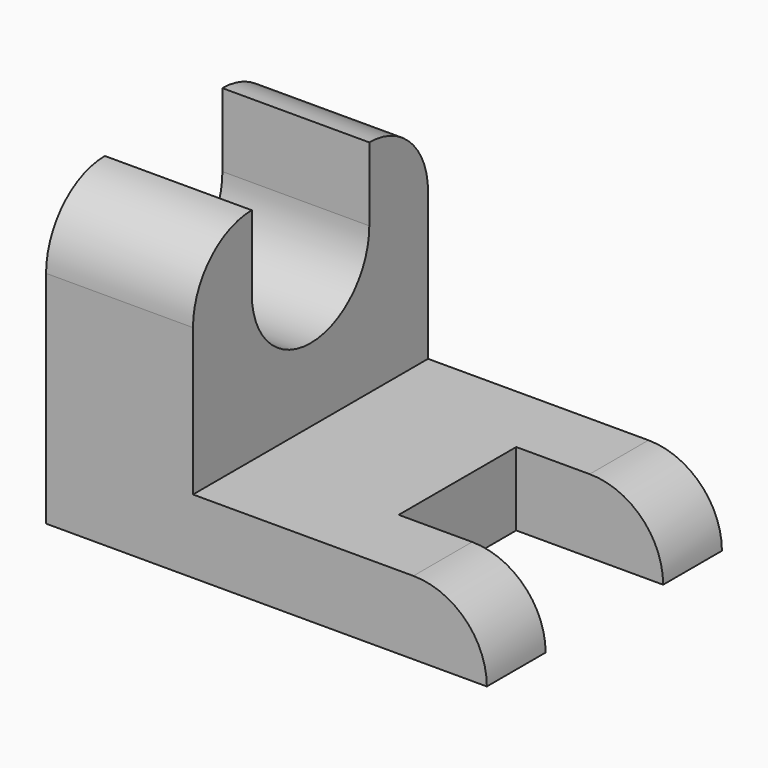
from build123d import *

# Parameters (mm, degrees)
F0_W     = 152.4
F0_H     = 101.6
F1_DEPTH = 25.4
F2_W     = 50.8
F2_H     = 50.8
F3_DEPTH = 25.401
F4_W     = 50.8
F4_H     = 101.6
F5_DEPTH = 76.2
F6_W     = 50.8
F6_H     = 25.4
F7_DEPTH = 50.801
F9_DEPTH = 50.801
F10_R    = 25.39999


# Not quite as in the source:
# - a fillet or chamfer is up to 0.001 mm smaller than in the source, because OpenCascade refuses the exact size


with BuildPart() as f1:
    # F0 (on Top) → F1 (new body)
    with BuildSketch(Plane.XY):
        with Locations((76.2, 50.8)):
            Rectangle(F0_W, F0_H)
    extrude(amount=F1_DEPTH)

    # F2 (on face) → F3 (cut, through all)
    with BuildSketch(Plane.XY.offset(25.4)):
        with Locations((127, 50.8)):
            Rectangle(F2_W, F2_H)
    extrude(amount=-F3_DEPTH, mode=Mode.SUBTRACT)

    # F4 (on face) → F5 (join)
    with BuildSketch(Plane.XY.offset(25.4)):
        with Locations((25.4, 50.8)):
            Rectangle(F4_W, F4_H)
    extrude(amount=F5_DEPTH)

    # F6 (on face) → F7 (cut, through all)
    with BuildSketch(Plane.YZ.offset(50.8)):
        with Locations((50.8, 88.9)):
            Rectangle(F6_W, F6_H)
    extrude(amount=-F7_DEPTH, mode=Mode.SUBTRACT)

    # F8 (on face) → F9 (cut, through all)
    with BuildSketch(Plane.YZ.offset(50.8)):
        with BuildLine():
            Line((76.2, 76.2), (25.4, 76.2))
            ThreePointArc((25.4, 76.2), (50.8, 50.8), (76.2, 76.2))
        make_face()
    extrude(amount=-F9_DEPTH, mode=Mode.SUBTRACT)

    # F10 (radius 25.4 in the source; OpenCascade refuses exactly that, so slightly less here)
    f10_edges = [f1.edges().sort_by_distance(p)[0] for p in [
        (25.4, 0, 101.6),
        (25.4, 101.6, 101.6),
        (152.4, 12.7, 25.4),
        (152.4, 88.9, 25.4),
    ]]
    fillet(f10_edges, radius=F10_R)


solid = f1.part
